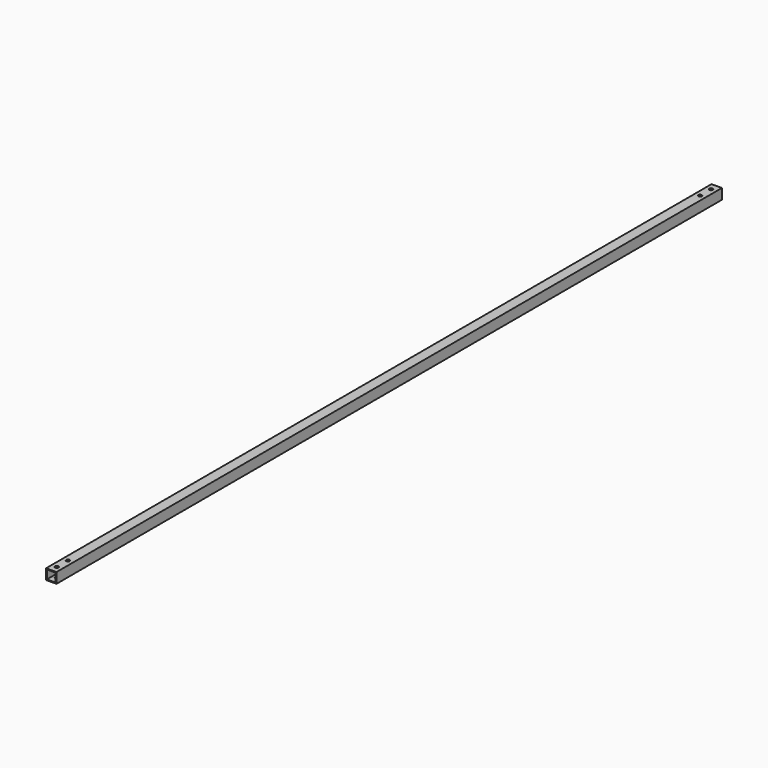
from build123d import *

# Parameters (mm, degrees)
F0_W     = 38.1
F0_H     = 38.1
F0_W_2   = 31.75
F0_H_2   = 31.75
F1_DEPTH = 3048
F2_R     = 6.35
F3_DEPTH = 38.101


# Not quite as in the source:
# - a feature names something its author has since deleted; it is built from what else it names


with BuildPart() as f1:
    # F0 (on Front) → F1 (new body)
    with BuildSketch(Plane.XZ):
        Rectangle(F0_W, F0_H)
        Rectangle(F0_W_2, F0_H_2, mode=Mode.SUBTRACT)
    extrude(amount=F1_DEPTH)

    # F2 (on face) → F3 (cut, through all)
    with BuildSketch(Plane.XY.offset(19.05)):
        with Locations((0, -25.4)):
            Circle(F2_R)
        with Locations((0, -76.2)):
            Circle(F2_R)
        with Locations((0, -3022.6)):
            Circle(F2_R)
        with Locations((0, -2971.8)):
            Circle(F2_R)
    extrude(amount=-F3_DEPTH, mode=Mode.SUBTRACT)


solid = f1.part
